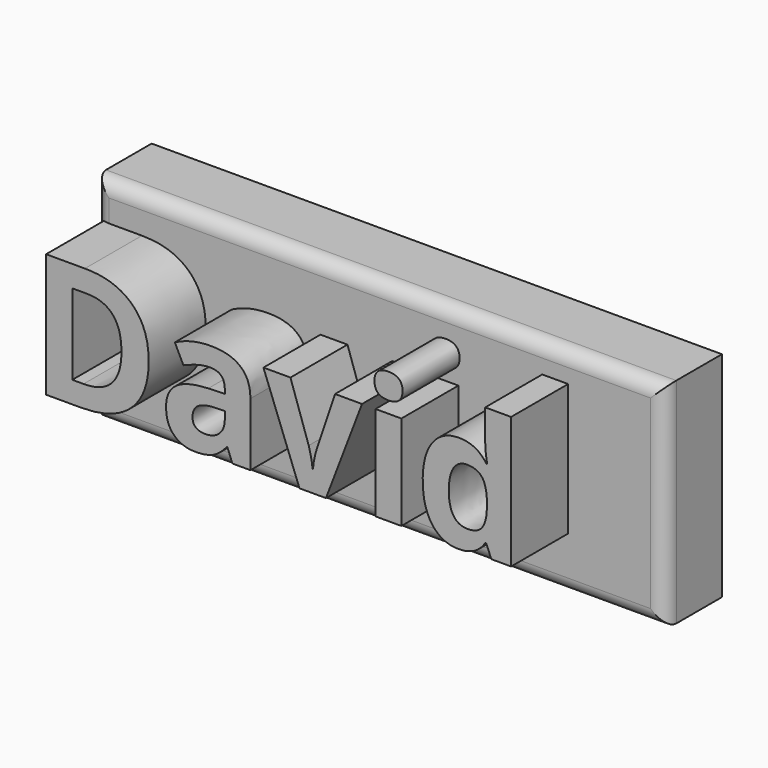
from build123d import *

# Parameters (mm, degrees)
F0_W         = 203.2
F0_H         = 76.2
F1_DEPTH     = 25.4
F2_R         = 5.08
F3_TEXT_SIZE = 61.7361111111
F4_DEPTH     = 50.8


# Not quite as in the source:
# - Text() gives the source's letters only with a copy of the font that has no kerning and outlines rounded to 1/6400 em; it was checked with that copy


with BuildPart() as f1:
    # F0 (on Front) → F1 (new body)
    with BuildSketch(Plane.XZ):
        with Locations((-7.9092432687, 3.8109850138)):
            Rectangle(F0_W, F0_H)
    extrude(amount=F1_DEPTH)

    # F2
    f2_edges = [f1.edges().sort_by_distance(p)[0] for p in [
        (-7.909243, -25.4, 41.910985),
        (-109.509243, -25.4, 3.810985),
        (-7.909243, -25.4, -34.289015),
        (93.690757, -25.4, 3.810985),
    ]]
    fillet(f2_edges, radius=F2_R)

    # F3 (on Front) → F4 (join)
    with BuildSketch(Plane.XZ):
        with Locations((-112.0233361506, -15.2390149862)):
            Text('David', F3_TEXT_SIZE, font='Open Sans', font_style=FontStyle.BOLD, text_align=(TextAlign.LEFT, TextAlign.BOTTOM))
    extrude(amount=F4_DEPTH)


solid = f1.part
